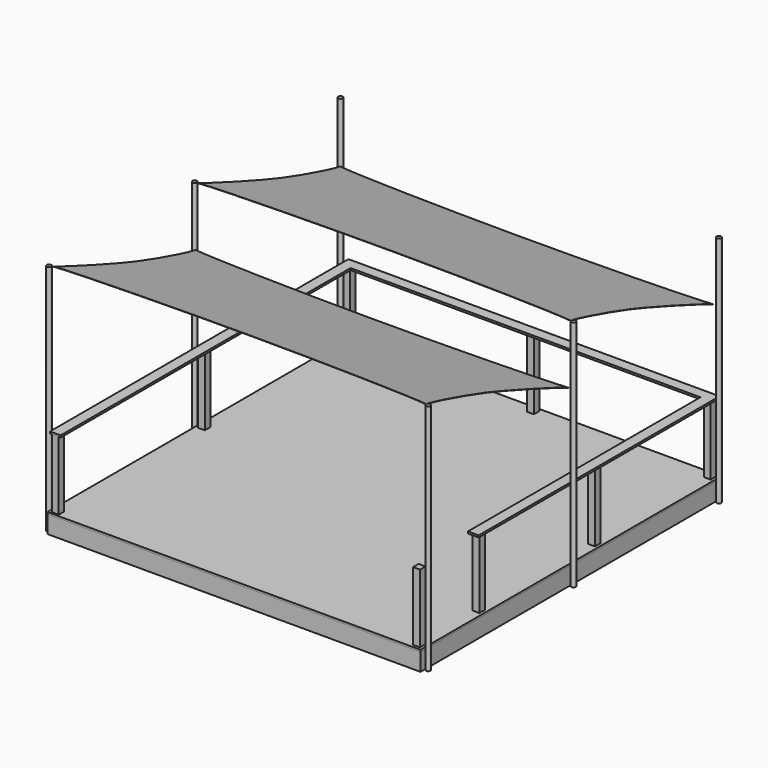
from build123d import *

# Parameters (mm, degrees)
F0_W      = 4876.8
F0_H      = 4914.9
F1_DEPTH  = 25.4
F2_W      = 4876.8
F2_H      = 4914.9
F2_W_2    = 4800.6
F2_H_2    = 4838.7
F3_DEPTH  = 228.6
F4_W      = 88.9
F4_H      = 88.9
F5_DEPTH  = 1149.35
F7_DEPTH  = 25.4
F8_R      = 30.1625
F9_DEPTH  = 3048
F13_DEPTH = 3.175


# Not quite as in the source:
# - the program builds the solid bodies; features that only make, move or delete a surface that nothing else refers to are left out


with BuildPart() as f1:
    # F0 (on Top) → F1 (new body)
    with BuildSketch(Plane.XY):
        Rectangle(F0_W, F0_H)
    extrude(amount=-F1_DEPTH)


with BuildPart() as f3:
    # F2 (on face) → F3 (new body)
    with BuildSketch(Plane(origin=(0, 0, -25.4), x_dir=(1, 0, 0), z_dir=(0, 0, -1))):
        Rectangle(F2_W, F2_H)
        Rectangle(F2_W_2, F2_H_2, mode=Mode.SUBTRACT)
    extrude(amount=F3_DEPTH)


with BuildPart() as f5:
    # F4 (on face) → F5 (new body)
    with BuildSketch(Plane(origin=(0, 0, -254), x_dir=(1, 0, 0), z_dir=(0, 0, -1))):
        with Locations((-2355.85, 2387.6)):
            Rectangle(F4_W, F4_H)
    extrude(amount=-F5_DEPTH)


with BuildPart() as f5b:
    # F4 (on face) → F5, piece 2 (new body)
    with BuildSketch(Plane(origin=(0, 0, -254), x_dir=(1, 0, 0), z_dir=(0, 0, -1))):
        with Locations((2355.85, 2374.9)):
            Rectangle(F4_W, F4_H)
    extrude(amount=-F5_DEPTH)


with BuildPart() as f5c:
    # F4 (on face) → F5, piece 3 (new body)
    with BuildSketch(Plane(origin=(0, 0, -254), x_dir=(1, 0, 0), z_dir=(0, 0, -1))):
        with Locations((44.45, -2374.9)):
            Rectangle(F4_W, F4_H)
    extrude(amount=-F5_DEPTH)


with BuildPart() as f5d:
    # F4 (on face) → F5, piece 4 (new body)
    with BuildSketch(Plane(origin=(0, 0, -254), x_dir=(1, 0, 0), z_dir=(0, 0, -1))):
        with Locations((-2355.85, -2374.9)):
            Rectangle(F4_W, F4_H)
    extrude(amount=-F5_DEPTH)


with BuildPart() as f5e:
    # F4 (on face) → F5, piece 5 (new body)
    with BuildSketch(Plane(origin=(0, 0, -254), x_dir=(1, 0, 0), z_dir=(0, 0, -1))):
        with Locations((-2355.85, 0)):
            Rectangle(F4_W, F4_H)
    extrude(amount=-F5_DEPTH)


with BuildPart() as f5f:
    # F4 (on face) → F5, piece 6 (new body)
    with BuildSketch(Plane(origin=(0, 0, -254), x_dir=(1, 0, 0), z_dir=(0, 0, -1))):
        with Locations((2355.85, -2374.9)):
            Rectangle(F4_W, F4_H)
    extrude(amount=-F5_DEPTH)


with BuildPart() as f5g:
    # F4 (on face) → F5, piece 7 (new body)
    with BuildSketch(Plane(origin=(0, 0, -254), x_dir=(1, 0, 0), z_dir=(0, 0, -1))):
        with Locations((2355.85, -482.6)):
            Rectangle(F4_W, F4_H)
    extrude(amount=-F5_DEPTH)


with BuildPart() as f5h:
    # F4 (on face) → F5, piece 8 (new body)
    with BuildSketch(Plane(origin=(0, 0, -254), x_dir=(1, 0, 0), z_dir=(0, 0, -1))):
        with Locations((2355.85, 1403.35)):
            Rectangle(F4_W, F4_H)
    extrude(amount=-F5_DEPTH)


with BuildPart() as f7:
    # F6 (on face) → F7 (new body)
    with BuildSketch(Plane.XY.offset(895.35)):
        Polygon((-2425.7, -2432.05), (-2286, -2432.05), (-2286, 2305.05), (2286, 2305.05), (2286, -1492.25), (2425.7, -1492.25), (2425.7, 2444.75), (-2425.7, 2444.75), align=None)
    extrude(amount=F7_DEPTH)


with BuildPart() as f9:
    # F8 (on face) → F9 (new body)
    with BuildSketch(Plane(origin=(0, 0, -254), x_dir=(1, 0, 0), z_dir=(0, 0, -1))):
        with Locations((-2473.325, -2374.9)):
            Circle(F8_R)
    extrude(amount=-F9_DEPTH)


with BuildPart() as f9b:
    # F8 (on face) → F9, piece 2 (new body)
    with BuildSketch(Plane(origin=(0, 0, -254), x_dir=(1, 0, 0), z_dir=(0, 0, -1))):
        with Locations((2473.325, -2374.9)):
            Circle(F8_R)
    extrude(amount=-F9_DEPTH)


with BuildPart() as f9c:
    # F8 (on face) → F9, piece 3 (new body)
    with BuildSketch(Plane(origin=(0, 0, -254), x_dir=(1, 0, 0), z_dir=(0, 0, -1))):
        with Locations((2473.325, 2374.9)):
            Circle(F8_R)
    extrude(amount=-F9_DEPTH)


with BuildPart() as f9d:
    # F8 (on face) → F9, piece 4 (new body)
    with BuildSketch(Plane(origin=(0, 0, -254), x_dir=(1, 0, 0), z_dir=(0, 0, -1))):
        with Locations((-2473.325, 2387.6)):
            Circle(F8_R)
    extrude(amount=-F9_DEPTH)


with BuildPart() as f9e:
    # F8 (on face) → F9, piece 5 (new body)
    with BuildSketch(Plane(origin=(0, 0, -254), x_dir=(1, 0, 0), z_dir=(0, 0, -1))):
        with Locations((-2473.325, 6.35)):
            Circle(F8_R)
    extrude(amount=-F9_DEPTH)


with BuildPart() as f9f:
    # F8 (on face) → F9, piece 6 (new body)
    with BuildSketch(Plane(origin=(0, 0, -254), x_dir=(1, 0, 0), z_dir=(0, 0, -1))):
        with Locations((2473.325, 0)):
            Circle(F8_R)
    extrude(amount=-F9_DEPTH)


with BuildPart() as f13:
    # F12 (on face) → F13 (new body)
    with BuildSketch(Plane(origin=(0, 817.5436775701, 2519.3422912103), x_dir=(1, 0, 0), z_dir=(0, 0.308661731, 0.951171875))):
        with BuildLine():
            add(Edge.make_bspline(
                [(2438.4, -859.5120388417), (2139.6498680115, -786.2739154141), (926.3832478326, -732.5120388417), (0, -732.5120388417)],
                knots=[0, 0, 0, 0, 2441.7050518029, 2441.7050518029, 2441.7050518029, 2441.7050518029], degree=3))
            add(Edge.make_bspline(
                [(2438.4, -859.5120388417), (2389.7120952606, -747.204382066), (2311.4, -21.9441822458), (2311.4, 359.6879611583)],
                knots=[0, 0, 0, 0, 1225.7967368206, 1225.7967368206, 1225.7967368206, 1225.7967368206], degree=3))
            add(Edge.make_bspline(
                [(2438.4, 1578.8879611583), (2389.7120952606, 1466.5803043826), (2311.4, 741.3201045624), (2311.4, 359.6879611583)],
                knots=[0, 0, 0, 0, 1225.7967368206, 1225.7967368206, 1225.7967368206, 1225.7967368206], degree=3))
            add(Edge.make_bspline(
                [(2438.4, 1578.8879611583), (2139.6498680115, 1505.6498377307), (926.3832478326, 1451.8879611583), (0, 1451.8879611583)],
                knots=[0, 0, 0, 0, 2441.7050518029, 2441.7050518029, 2441.7050518029, 2441.7050518029], degree=3))
            add(Edge.make_bspline(
                [(-2438.4, 1578.8879611583), (-2139.6498680115, 1505.6498377307), (-926.3832478326, 1451.8879611583), (0, 1451.8879611583)],
                knots=[0, 0, 0, 0, 2441.7050518029, 2441.7050518029, 2441.7050518029, 2441.7050518029], degree=3))
            add(Edge.make_bspline(
                [(-2438.4, 1578.8879611583), (-2389.7120952606, 1466.5803043826), (-2311.4, 741.3201045624), (-2311.4, 359.6879611583)],
                knots=[0, 0, 0, 0, 1225.7967368206, 1225.7967368206, 1225.7967368206, 1225.7967368206], degree=3))
            add(Edge.make_bspline(
                [(-2438.4, -859.5120388417), (-2389.7120952606, -747.204382066), (-2311.4, -21.9441822458), (-2311.4, 359.6879611583)],
                knots=[0, 0, 0, 0, 1225.7967368206, 1225.7967368206, 1225.7967368206, 1225.7967368206], degree=3))
            add(Edge.make_bspline(
                [(-2438.4, -859.5120388417), (-2139.6498680115, -786.2739154141), (-926.3832478326, -732.5120388417), (0, -732.5120388417)],
                knots=[0, 0, 0, 0, 2441.7050518029, 2441.7050518029, 2441.7050518029, 2441.7050518029], degree=3))
        make_face()
    extrude(amount=F13_DEPTH)


with BuildPart() as f14_1:
    # F14: copy of F13
    add(f13.part.moved(Location((0, -2362.2, 0))))


solid = Compound([f1.part, f3.part, f5.part, f5b.part, f5c.part, f5d.part, f5e.part, f5f.part, f5g.part, f5h.part, f7.part, f9.part, f9b.part, f9c.part, f9d.part, f9e.part, f9f.part, f13.part, f14_1.part])
